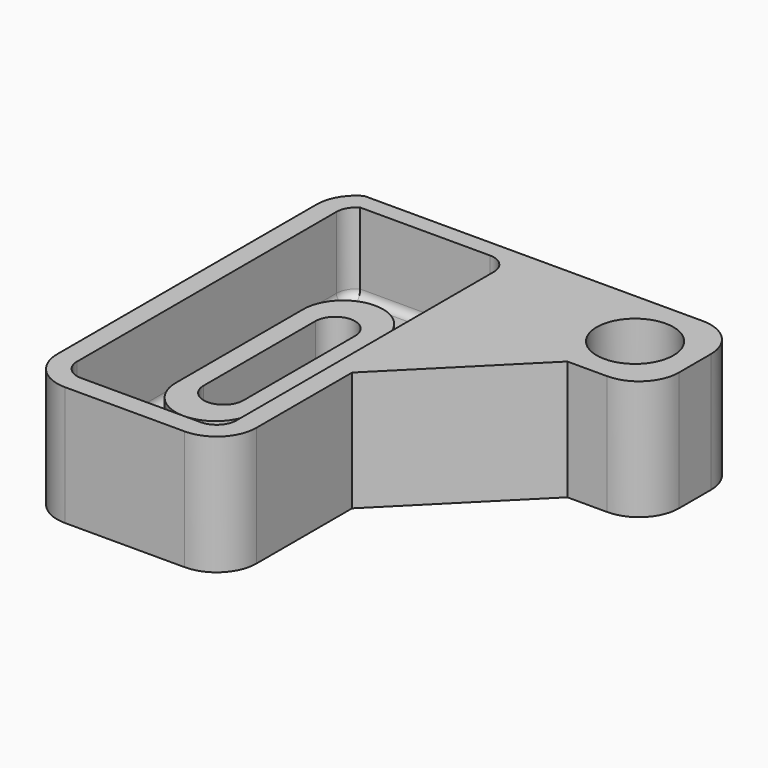
from build123d import *

# Parameters (mm, degrees)
F1_DEPTH       = 30
F3_D           = 12.6
F3_CBORE_D     = 19.25
F3_CBORE_DEPTH = 12
F5_DEPTH       = 20
F7_DEPTH       = 10
F9_T1_DEPTH    = 80.6698729811
F9_T3_DEPTH    = 37.5
F9_T5_DEPTH    = 30
F9_T7_DEPTH    = 81.3397459622
F9_T9_DEPTH    = 40
F9_T12_ANGLE   = 90
F9_T14_ANGLE   = 90
F9_T16_ANGLE   = 117.3060073295
F9_T18_ANGLE   = 90
F9_T20_ANGLE   = 180
F9_T22_ANGLE   = 180
F10_DEPTH      = 20.001


# Not quite as in the source:
# - a fillet or chamfer that OpenCascade refuses, or shapes differently, is made with other operations: its cross-section is extruded or revolved along the edge and cut away or added


with BuildPart() as f1:
    # F0 (on Top) → F1 (new body)
    with BuildSketch(Plane.XY):
        with BuildLine():
            Line((0, -30), (0, 0))
            Line((0, 0), (30, 30))
            Line((30, 30), (40, 30))
            ThreePointArc((40, 30), (47.0710678119, 32.9289321881), (50, 40))
            Line((50, 40), (50, 50))
            ThreePointArc((50, 50), (47.0710678119, 57.0710678119), (40, 60))
            Line((40, 60), (-45, 60))
            ThreePointArc((-45, 60), (-48.6602540378, 56.3397459622), (-50, 51.3397459622))
            Line((-50, 51.3397459622), (-50, -30))
            ThreePointArc((-50, -30), (-47.0710678119, -37.0710678119), (-40, -40))
            Line((-40, -40), (-10, -40))
            ThreePointArc((-10, -40), (-2.9289321881, -37.0710678119), (0, -30))
        make_face()
    extrude(amount=F1_DEPTH)

    # F3 (through all)
    with Locations(Plane.XY.offset(30)):
        with Locations((35, 45)):
            CounterBoreHole(F3_D / 2, F3_CBORE_D / 2, F3_CBORE_DEPTH)

    # F4 (on face) → F5 (cut)
    with BuildSketch(Plane.XY.offset(30)):
        with BuildLine():
            Line((-10, 55.6698729811), (-42.5, 55.6698729811))
            ThreePointArc((-42.5, 55.6698729811), (-44.3301270189, 53.8397459622), (-45, 51.3397459622))
            Line((-45, 51.3397459622), (-45, -30))
            ThreePointArc((-45, -30), (-43.5355339059, -33.5355339059), (-40, -35))
            Line((-40, -35), (-10, -35))
            ThreePointArc((-10, -35), (-6.4644660941, -33.5355339059), (-5, -30))
            Line((-5, -30), (-5, 50.6698729811))
            ThreePointArc((-5, 50.6698729811), (-6.4644660941, 54.205406887), (-10, 55.6698729811))
        make_face()
    extrude(amount=-F5_DEPTH, mode=Mode.SUBTRACT)

    # F6 (on face) → F7 (join)
    with BuildSketch(Plane.XY.offset(10)):
        with BuildLine():
            ThreePointArc((-16.25, 30), (-26.25, 40), (-36.25, 30))
            Line((-36.25, 30), (-36.25, -10))
            ThreePointArc((-36.25, -10), (-26.25, -20), (-16.25, -10))
            Line((-16.25, -10), (-16.25, 30))
        make_face()
    extrude(amount=F7_DEPTH)

    # F9: fillet of radius 2 on 12 edges, made by hand

    # F9_s2 → F9_t1 (join)
    with BuildSketch(Plane.XZ.offset(-50.6698729811)):
        with BuildLine():
            ThreePointArc((-5, 12), (-5.5857864376, 10.5857864376), (-7, 10))
            Line((-7, 10), (-5, 10))
            Line((-5, 10), (-5, 12))
        make_face()
    extrude(amount=F9_T1_DEPTH)

    # F9_s4 → F9_t3 (join)
    with BuildSketch(Plane.YZ.offset(-47.5)):
        with BuildLine():
            ThreePointArc((55.6698729811, 12), (55.0840865435, 10.5857864376), (53.6698729811, 10))
            Line((53.6698729811, 10), (55.6698729811, 10))
            Line((55.6698729811, 10), (55.6698729811, 12))
        make_face()
    extrude(amount=F9_T3_DEPTH)

    # F9_s6 → F9_t5 (join)
    with BuildSketch(Plane.YZ.offset(-40)):
        with BuildLine():
            ThreePointArc((-35, 12), (-34.4142135624, 10.5857864376), (-33, 10))
            Line((-33, 10), (-35, 10))
            Line((-35, 10), (-35, 12))
        make_face()
    extrude(amount=F9_T5_DEPTH)

    # F9_s8 → F9_t7 (join)
    with BuildSketch(Plane.XZ.offset(-51.3397459622)):
        with BuildLine():
            ThreePointArc((-45, 12), (-44.4142135624, 10.5857864376), (-43, 10))
            Line((-43, 10), (-45, 10))
            Line((-45, 10), (-45, 12))
        make_face()
    extrude(amount=F9_T7_DEPTH)

    # F9_s10 → F9_t9 (join)
    with BuildSketch(Plane.XZ.offset(-30)):
        with BuildLine():
            ThreePointArc((-14.25, 10), (-15.6642135624, 10.5857864376), (-16.25, 12))
            Line((-16.25, 12), (-16.25, 10))
            Line((-16.25, 10), (-14.25, 10))
        make_face()
        with BuildLine():
            ThreePointArc((-38.25, 10), (-36.8357864376, 10.5857864376), (-36.25, 12))
            Line((-36.25, 12), (-36.25, 10))
            Line((-36.25, 10), (-38.25, 10))
        make_face()
    extrude(amount=F9_T9_DEPTH)

    # F9_s11 → F9_t12 (revolve)
    with BuildSketch(Plane.XZ.offset(-50.6698729811)):
        with BuildLine():
            ThreePointArc((-5, 12), (-5.5857864376, 10.5857864376), (-7, 10))
            Line((-7, 10), (-5, 10))
            Line((-5, 10), (-5, 12))
        make_face()
    revolve(axis=Axis((-10, 50.6698729811, 10), (0, 0, 1)), revolution_arc=F9_T12_ANGLE)

    # F9_s13 → F9_t14 (revolve)
    with BuildSketch(Plane.YZ.offset(-10)):
        with BuildLine():
            ThreePointArc((-35, 12), (-34.4142135624, 10.5857864376), (-33, 10))
            Line((-33, 10), (-35, 10))
            Line((-35, 10), (-35, 12))
        make_face()
    revolve(axis=Axis((-10, -30, 10), (0, 0, 1)), revolution_arc=F9_T14_ANGLE)

    # F9_s15 → F9_t16 (revolve)
    with BuildSketch(Plane(origin=(-52.509549327, 27.1091719145, 0), x_dir=(0, 0, 1), z_dir=(0.8885691394, -0.4587427214, 0))):
        with BuildLine():
            ThreePointArc((12, -32.2692050314), (10.5857864376, -31.6834185938), (10, -30.2692050314))
            Line((10, -30.2692050314), (10, -32.2692050314))
            Line((10, -32.2692050314), (12, -32.2692050314))
        make_face()
    revolve(axis=Axis((-40, 51.3397459622, 10), (0, 0, 1)), revolution_arc=F9_T16_ANGLE)

    # F9_s17 → F9_t18 (revolve)
    with BuildSketch(Plane.XZ.offset(30)):
        with BuildLine():
            ThreePointArc((-45, 12), (-44.4142135624, 10.5857864376), (-43, 10))
            Line((-43, 10), (-45, 10))
            Line((-45, 10), (-45, 12))
        make_face()
    revolve(axis=Axis((-40, -30, 10), (0, 0, 1)), revolution_arc=F9_T18_ANGLE)

    # F9_s19 → F9_t20 (revolve)
    with BuildSketch(Plane.XZ.offset(10)):
        with BuildLine():
            ThreePointArc((-38.25, 10), (-36.8357864376, 10.5857864376), (-36.25, 12))
            Line((-36.25, 12), (-36.25, 10))
            Line((-36.25, 10), (-38.25, 10))
        make_face()
    revolve(axis=Axis((-26.25, -10, 10), (0, 0, 1)), revolution_arc=F9_T20_ANGLE)

    # F9_s21 → F9_t22 (revolve)
    with BuildSketch(Plane.XZ.offset(-30)):
        with BuildLine():
            ThreePointArc((-14.25, 10), (-15.6642135624, 10.5857864376), (-16.25, 12))
            Line((-16.25, 12), (-16.25, 10))
            Line((-16.25, 10), (-14.25, 10))
        make_face()
    revolve(axis=Axis((-26.25, 30, 10), (0, 0, 1)), revolution_arc=F9_T22_ANGLE)

    # F8 (on face) → F10 (cut, through all)
    with BuildSketch(Plane.XY.offset(20)):
        with BuildLine():
            ThreePointArc((-31.25, -7.5), (-26.25, -12.5), (-21.25, -7.5))
            Line((-21.25, -7.5), (-21.25, 27.5))
            ThreePointArc((-21.25, 27.5), (-26.25, 32.5), (-31.25, 27.5))
            Line((-31.25, 27.5), (-31.25, -7.5))
        make_face()
    extrude(amount=-F10_DEPTH, mode=Mode.SUBTRACT)


solid = f1.part
